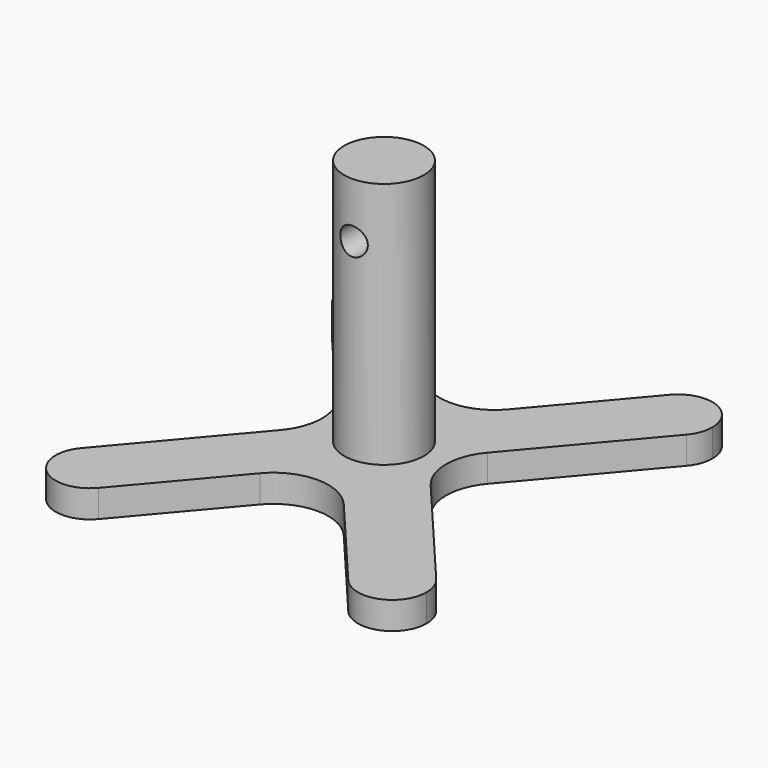
from build123d import *

# Parameters (mm, degrees)
F1_DEPTH = 10
F3_R     = 14.5
F4_DEPTH = 90
F2_R     = 5
F5_DEPTH = 25


# Not quite as in the source:
# - a feature names something its author has since deleted; it is built from what else it names


with BuildPart() as f1:
    # F0 (on Top) → F1 (new body)
    with BuildSketch(Plane.XY):
        with BuildLine():
            Line((-45.4576714329, 73.0742780183), (-55, 65))
            Line((-55, 65), (-46.9257219817, 55.4576714329))
            ThreePointArc((-46.9257219817, 55.4576714329), (-43.6602805319, 59.7406500035), (-42.5, 65))
            ThreePointArc((-42.5, 65), (-43.2626854202, 69.2994704855), (-45.4576714329, 73.0742780183))
        make_face()
        with BuildLine():
            Line((-46.9257219817, 55.4576714329), (-55, 65))
            Line((-55, 65), (-64.5423285671, 56.9257219817))
            ThreePointArc((-64.5423285671, 56.9257219817), (-56.0380684982, 52.5431780219), (-46.9257219817, 55.4576714329))
        make_face()
        with BuildLine():
            Line((-64.5423285671, 56.9257219817), (-55, 65))
            Line((-55, 65), (-45.4576714329, 73.0742780183))
            ThreePointArc((-45.4576714329, 73.0742780183), (-63.0742780183, 74.5423285671), (-64.5423285671, 56.9257219817))
        make_face()
        with BuildLine():
            ThreePointArc((-42.5, 65), (-43.6602805319, 59.7406500035), (-46.9257219817, 55.4576714329))
            Line((-46.9257219817, 55.4576714329), (-9.3661625013, 11.0691011379))
            ThreePointArc((-9.3661625013, 11.0691011379), (0, 14.5), (9.3661625013, 11.0691011379))
            Line((9.3661625013, 11.0691011379), (46.9257219817, 55.4576714329))
            ThreePointArc((46.9257219817, 55.4576714329), (42.5431780219, 63.9619315018), (45.4576714329, 73.0742780183))
            Line((45.4576714329, 73.0742780183), (15.2677257074, 37.3952512518))
            ThreePointArc((15.2677257074, 37.3952512518), (0, 30.3140960811), (-15.2677257074, 37.3952512518))
            Line((-15.2677257074, 37.3952512518), (-45.4576714329, 73.0742780183))
            ThreePointArc((-45.4576714329, 73.0742780183), (-43.2626854202, 69.2994704855), (-42.5, 65))
        make_face()
        with BuildLine():
            Line((-9.3661625013, 11.0691011379), (-46.9257219817, 55.4576714329))
            ThreePointArc((-46.9257219817, 55.4576714329), (-56.0380684982, 52.5431780219), (-64.5423285671, 56.9257219817))
            Line((-64.5423285671, 56.9257219817), (-27.3057402074, 12.9188448293))
            ThreePointArc((-27.3057402074, 12.9188448293), (-22.5734659148, 0), (-27.3057402074, -12.9188448293))
            Line((-27.3057402074, -12.9188448293), (-64.5423285671, -56.9257219817))
            ThreePointArc((-64.5423285671, -56.9257219817), (-56.0380684982, -52.5431780219), (-46.9257219817, -55.4576714329))
            Line((-46.9257219817, -55.4576714329), (-9.3661625013, -11.0691011379))
            ThreePointArc((-9.3661625013, -11.0691011379), (-14.5, 0), (-9.3661625013, 11.0691011379))
        make_face()
        with BuildLine():
            ThreePointArc((9.3661625013, 11.0691011379), (0, 14.5), (-9.3661625013, 11.0691011379))
            Line((-9.3661625013, 11.0691011379), (0, 0))
            Line((0, 0), (9.3661625013, 11.0691011379))
        make_face()
        with BuildLine():
            Line((0, 0), (-9.3661625013, 11.0691011379))
            ThreePointArc((-9.3661625013, 11.0691011379), (-14.5, 0), (-9.3661625013, -11.0691011379))
            Line((-9.3661625013, -11.0691011379), (0, 0))
        make_face()
        with BuildLine():
            Line((9.3661625013, 11.0691011379), (0, 0))
            Line((0, 0), (9.3661625013, -11.0691011379))
            ThreePointArc((9.3661625013, -11.0691011379), (13.154074583, -6.1008459959), (14.5, 0))
            ThreePointArc((14.5, 0), (13.154074583, 6.1008459959), (9.3661625013, 11.0691011379))
        make_face()
        with BuildLine():
            Line((9.3661625013, -11.0691011379), (0, 0))
            Line((0, 0), (-9.3661625013, -11.0691011379))
            ThreePointArc((-9.3661625013, -11.0691011379), (0, -14.5), (9.3661625013, -11.0691011379))
        make_face()
        with BuildLine():
            Line((46.9257219817, 55.4576714329), (9.3661625013, 11.0691011379))
            ThreePointArc((9.3661625013, 11.0691011379), (13.154074583, 6.1008459959), (14.5, 0))
            ThreePointArc((14.5, 0), (13.154074583, -6.1008459959), (9.3661625013, -11.0691011379))
            Line((9.3661625013, -11.0691011379), (46.9257219817, -55.4576714329))
            ThreePointArc((46.9257219817, -55.4576714329), (56.0380684982, -52.5431780219), (64.5423285671, -56.9257219817))
            Line((64.5423285671, -56.9257219817), (27.3057402074, -12.9188448293))
            ThreePointArc((27.3057402074, -12.9188448293), (22.5734659148, 0), (27.3057402074, 12.9188448293))
            Line((27.3057402074, 12.9188448293), (64.5423285671, 56.9257219817))
            ThreePointArc((64.5423285671, 56.9257219817), (56.0380684982, 52.5431780219), (46.9257219817, 55.4576714329))
        make_face()
        with BuildLine():
            ThreePointArc((9.3661625013, -11.0691011379), (0, -14.5), (-9.3661625013, -11.0691011379))
            Line((-9.3661625013, -11.0691011379), (-46.9257219817, -55.4576714329))
            ThreePointArc((-46.9257219817, -55.4576714329), (-43.6602805319, -59.7406500035), (-42.5, -65))
            ThreePointArc((-42.5, -65), (-43.2626854202, -69.2994704855), (-45.4576714329, -73.0742780183))
            Line((-45.4576714329, -73.0742780183), (-15.2677257074, -37.3952512518))
            ThreePointArc((-15.2677257074, -37.3952512518), (0, -30.3140960811), (15.2677257074, -37.3952512518))
            Line((15.2677257074, -37.3952512518), (45.4576714329, -73.0742780183))
            ThreePointArc((45.4576714329, -73.0742780183), (42.5431780219, -63.9619315018), (46.9257219817, -55.4576714329))
            Line((46.9257219817, -55.4576714329), (9.3661625013, -11.0691011379))
        make_face()
        with BuildLine():
            ThreePointArc((45.4576714329, 73.0742780183), (42.5431780219, 63.9619315018), (46.9257219817, 55.4576714329))
            Line((46.9257219817, 55.4576714329), (55, 65))
            Line((55, 65), (45.4576714329, 73.0742780183))
        make_face()
        with BuildLine():
            Line((55, 65), (46.9257219817, 55.4576714329))
            ThreePointArc((46.9257219817, 55.4576714329), (56.0380684982, 52.5431780219), (64.5423285671, 56.9257219817))
            Line((64.5423285671, 56.9257219817), (55, 65))
        make_face()
        with BuildLine():
            ThreePointArc((-42.5, -65), (-43.6602805319, -59.7406500035), (-46.9257219817, -55.4576714329))
            Line((-46.9257219817, -55.4576714329), (-55, -65))
            Line((-55, -65), (-45.4576714329, -73.0742780183))
            ThreePointArc((-45.4576714329, -73.0742780183), (-43.2626854202, -69.2994704855), (-42.5, -65))
        make_face()
        with BuildLine():
            Line((-55, -65), (-46.9257219817, -55.4576714329))
            ThreePointArc((-46.9257219817, -55.4576714329), (-56.0380684982, -52.5431780219), (-64.5423285671, -56.9257219817))
            Line((-64.5423285671, -56.9257219817), (-55, -65))
        make_face()
        with BuildLine():
            Line((-55, -65), (-64.5423285671, -56.9257219817))
            ThreePointArc((-64.5423285671, -56.9257219817), (-63.0742780183, -74.5423285671), (-45.4576714329, -73.0742780183))
            Line((-45.4576714329, -73.0742780183), (-55, -65))
        make_face()
        with BuildLine():
            ThreePointArc((67.5, 65), (59.2994704855, 76.7373145798), (45.4576714329, 73.0742780183))
            Line((45.4576714329, 73.0742780183), (55, 65))
            Line((55, 65), (64.5423285671, 56.9257219817))
            ThreePointArc((64.5423285671, 56.9257219817), (66.7373145798, 60.7005295145), (67.5, 65))
        make_face()
        with BuildLine():
            ThreePointArc((64.5423285671, -56.9257219817), (56.0380684982, -52.5431780219), (46.9257219817, -55.4576714329))
            Line((46.9257219817, -55.4576714329), (55, -65))
            Line((55, -65), (64.5423285671, -56.9257219817))
        make_face()
        with BuildLine():
            Line((55, -65), (46.9257219817, -55.4576714329))
            ThreePointArc((46.9257219817, -55.4576714329), (42.5431780219, -63.9619315018), (45.4576714329, -73.0742780183))
            Line((45.4576714329, -73.0742780183), (55, -65))
        make_face()
        with BuildLine():
            Line((64.5423285671, -56.9257219817), (55, -65))
            Line((55, -65), (45.4576714329, -73.0742780183))
            ThreePointArc((45.4576714329, -73.0742780183), (59.2994704855, -76.7373145798), (67.5, -65))
            ThreePointArc((67.5, -65), (66.7373145798, -60.7005295145), (64.5423285671, -56.9257219817))
        make_face()
    extrude(amount=F1_DEPTH)

    # F3 (on face) → F4 (join)
    with BuildSketch(Plane.XY.offset(10)):
        Circle(F3_R)
    extrude(amount=F4_DEPTH)

    # F2 (on Front) → F5 (cut, symmetric)
    with BuildSketch(Plane.XZ):
        with Locations((0, 80)):
            Circle(F2_R)
    extrude(amount=F5_DEPTH, both=True, mode=Mode.SUBTRACT)


solid = f1.part
